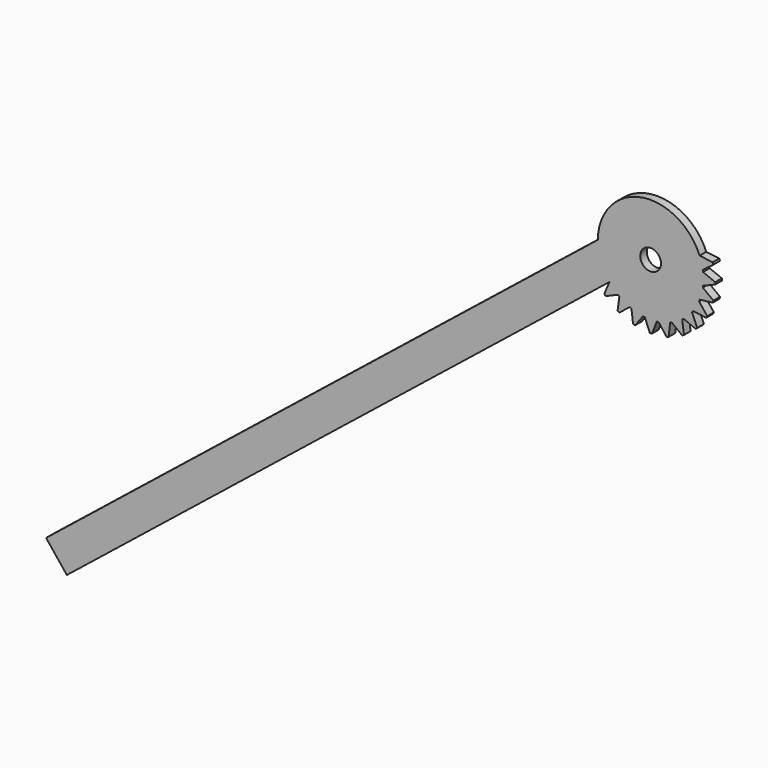
from build123d import *

# Parameters (mm, degrees)
F1_DEPTH        = 5
F2_DEPTH        = 5
F2_COPIES_COUNT = 11
F2_COPIES_ANGLE = 150
F3_R            = 12.5
F4_DEPTH        = 10.001


# Not quite as in the source:
# - a pattern or mirror of a feature is missing from the dataset's text; its kind, count and spacing are read off the source's solid


with BuildPart() as f1:
    # F0 (on Front) → F1 (new body, symmetric)
    with BuildSketch(Plane.XZ):
        with BuildLine():
            Line((-25.0008701164, 31.2242933215), (-63.4987428752, 0.3995663471))
            ThreePointArc((-63.4987428752, 0.3995663471), (-59.9818720369, -20.842865133), (-49.5685656478, -39.6888813097))
            Line((-49.5685656478, -39.6888813097), (0, 0))
            Line((0, 0), (-25.0008701164, 31.2242933215))
        make_face()
        with BuildLine():
            Line((0, 0), (62.772077735, 9.5872966381))
            ThreePointArc((62.772077735, 9.5872966381), (-4.6082108818, 63.3325697605), (-63.4987428752, 0.3995663471))
            Line((-63.4987428752, 0.3995663471), (-25.0008701164, 31.2242933215))
            Line((-25.0008701164, 31.2242933215), (0, 0))
        make_face()
        with BuildLine():
            ThreePointArc((-39.3237135407, -49.8587560351), (27.705542678, -57.1371412036), (63.5, 0))
            ThreePointArc((63.5, 0), (63.3177579206, 4.8074454664), (62.772077735, 9.5872966381))
            Line((62.772077735, 9.5872966381), (0, 0))
            Line((0, 0), (-49.5685656478, -39.6888813097))
            ThreePointArc((-49.5685656478, -39.6888813097), (-44.7360694833, -45.065886069), (-39.3237135407, -49.8587560351))
        make_face()
        with BuildLine():
            ThreePointArc((-49.5685656478, -39.6888813097), (-59.9818720369, -20.842865133), (-63.4987428752, 0.3995663471))
            Line((-63.4987428752, 0.3995663471), (-727.5474698493, -531.2952842967))
            Line((-727.5474698493, -531.2952842967), (-702.5465997329, -562.5195776181))
            Line((-702.5465997329, -562.5195776181), (-49.5685656478, -39.6888813097))
        make_face()
    extrude(amount=F1_DEPTH, both=True)

    # F0 (on Front) → F2 (join, symmetric)
    with BuildSketch(Plane.XZ):
        with BuildLine():
            Line((-53.9442142409, -56.1162132047), (-39.3237135407, -49.8587560351))
            ThreePointArc((-39.3237135407, -49.8587560351), (-44.7360694833, -45.065886069), (-49.5685656478, -39.6888813097))
            Line((-49.5685656478, -39.6888813097), (-55.718461724, -54.3549506266))
            Line((-55.718461724, -54.3549506266), (-53.9442142409, -56.1162132047))
        make_face()
    f2 = extrude(amount=F2_DEPTH, both=True)

    # F2_copies: F2 ×11 about axis
    f2_copies_axis = Axis((0, 0, 0), (0, -1, 0))
    for i in range(1, F2_COPIES_COUNT):
        add(f2.rotate(f2_copies_axis, i * F2_COPIES_ANGLE / (F2_COPIES_COUNT - 1)))

    # F3 (on face) → F4 (cut, through all)
    with BuildSketch(Plane(origin=(0, 5, 0), x_dir=(-1, 0, 0), z_dir=(0, 1, 0))):
        Circle(F3_R)
    extrude(amount=-F4_DEPTH, mode=Mode.SUBTRACT)


solid = f1.part
